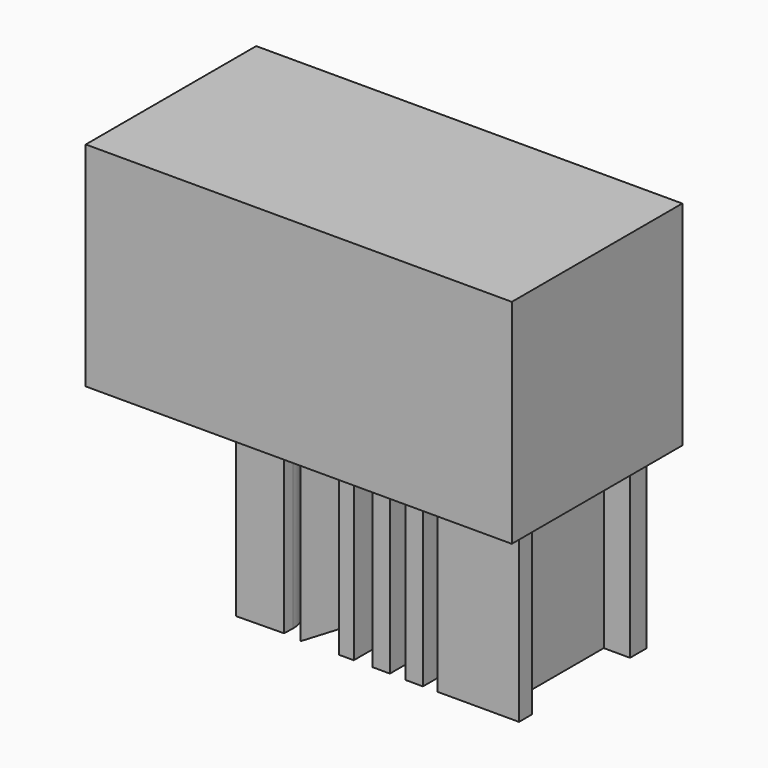
from build123d import *

# Parameters (mm, degrees)
F1_W     = 82.55
F1_H     = 82.55
F2_DEPTH = 41.275
F3_DEPTH = 82.55
F4_W     = 6.6821798682
F4_H     = 53.7756439298
F4_H_2   = 29.7516137362
F4_R     = 3.7333162537
F5_DEPTH = 67.31


# Not quite as in the source:
# - a variable given as a bare number and used for a length is read in inches; the dataset says mm whatever the document's units were


with BuildPart() as f2:
    # F1 (on Top) → F2 (new body, symmetric)
    with BuildSketch(Plane.XY):
        Rectangle(F1_W, F1_H)
    extrude(amount=F2_DEPTH, both=True)

    # F3 (add): a face of the model
    f3_faces = [f2.faces().sort_by_distance(p)[0] for p in [
        (41.275, 0, 0),
    ]]
    extrude(f3_faces, amount=F3_DEPTH)

    # F4 (on face) → F5 (join)
    with BuildSketch(Plane(origin=(0, 0, -41.275), x_dir=(1, 0, 0), z_dir=(0, 0, -1))):
        Polygon((117.642775178, -23.7058307976), (107.4604094028, -23.7058307976), (107.4604094028, 23.7058326602), (117.642775178, 23.7058326602), (117.642775178, 30.0698131323), (86.1410722136, 30.0698131323), (86.1410722136, 23.7058326602), (98.2326343656, 23.7058326602), (98.2326343656, -23.7058307976), (86.1410722136, -23.7058307976), (86.1410722136, -31.6608063877), (117.642775178, -31.6608063877), align=None)
        with Locations((77.0723931491, 3.1819911674)):
            Rectangle(F4_W, F4_H)
        with Locations((64.0262328088, 14.8758068681)):
            Rectangle(F4_W, F4_H_2)
        Polygon((60.6851428747, -10.9778670594), (67.3673227429, -11.2960664555), (67.3673227429, -3.9774877951), (60.6851428747, -3.9774877951), align=None)
        with BuildLine():
            Line((47.6389825344, 0), (53.3665642142, 0))
            Line((53.3665642142, 0), (53.3665642142, 29.7516137362))
            Line((53.3665642142, 29.7516137362), (47.6389825344, 29.7516137362))
            Line((47.6389825344, 29.7516137362), (39.7581494696, 8.1140771508))
            Line((39.7581494696, 8.1140771508), (33.0018214881, 30.0698131323))
            Line((33.0018214881, 30.0698131323), (33.0018214881, 4.0570385754))
            ThreePointArc((33.0018214881, 4.0570385754), (41.8631479069, 0.5195718098), (47.6389825344, 8.1140771508))
            Line((47.6389825344, 8.1140771508), (47.6389825344, 0))
        make_face()
        with BuildLine():
            ThreePointArc((7.5458958745, 29.43341434), (6.649165746, 16.0704833991), (11.6824880242, 3.6592902616))
            ThreePointArc((11.6824880242, 3.6592902616), (19.7418824044, 0.862989669), (28.2288361341, 0))
            Line((28.2288361341, 0), (28.2288361341, 6.8412809633))
            ThreePointArc((28.2288361341, 6.8412809633), (19.3054549337, 7.9595465035), (12.0006818324, 13.2052628323))
            ThreePointArc((12.0006818324, 13.2052628323), (21.7952321918, 15.7282111285), (25.9655225304, 24.9427194354))
            Line((25.9655225304, 24.9427194354), (25.8736382976, 29.1471914205))
            Line((25.8736382976, 29.1471914205), (7.5458958745, 29.43341434))
        make_face()
        with Locations((15.6531465528, 21.2212410615)):
            Circle(F4_R, mode=Mode.SUBTRACT)
    extrude(amount=F5_DEPTH)


solid = f2.part
